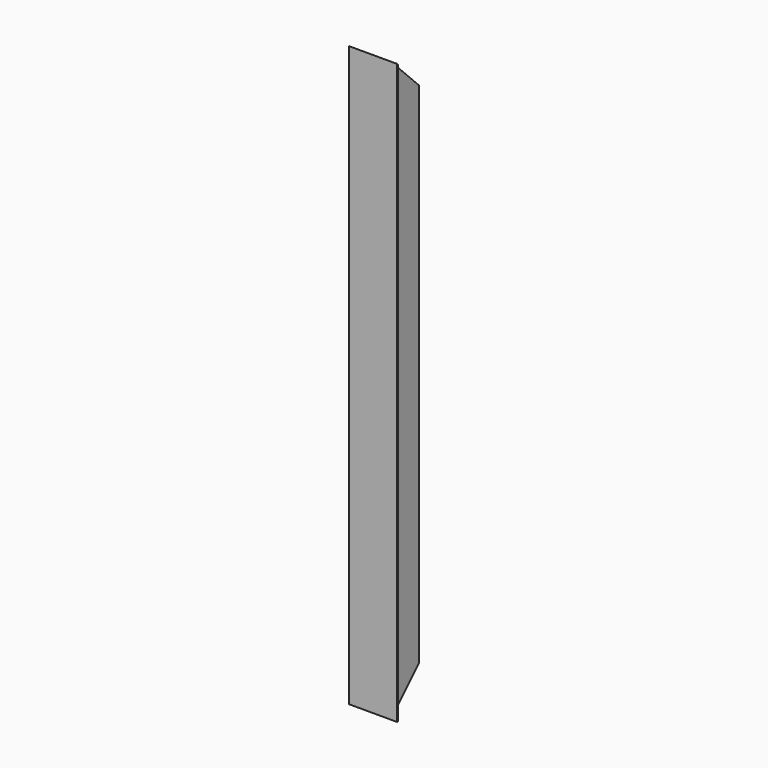
from build123d import *

# Parameters (mm, degrees)
F1_DEPTH = 228
F3_DEPTH = 30
F4_R     = 1
F6_R     = 0.5
F7_R     = 0.5


# Not quite as in the source:
# - two fillets or chamfers of one size are made in one step
# - a pattern or mirror of a feature is missing from the dataset's text; its kind, count and spacing are read off the source's solid


with BuildPart() as f1:
    # F0 (on Top) → F1 (new body, symmetric)
    with BuildSketch(Plane.XY):
        Polygon((-14, 0.5), (-17, 0.5), (-20, -2.5), (20, -2.5), (17, 0.5), (14, 0.5), (11, 0.5), (-11, 0.5), align=None)
        Polygon((-14, 25.5), (-14, 0.5), (-11, 0.5), (-11, 4), (-11, 7), (-11, 25.5), align=None)
        Polygon((11, 4), (11, 0.5), (14, 0.5), (14, 25.5), (11, 25.5), (11, 7), align=None)
        Polygon((-11, 7), (-11, 4), (-5, 4), (-5, 7), (-5, 15), (-8, 15), (-8, 7), align=None)
        Polygon((5, 4), (11, 4), (11, 7), (8, 7), (8, 15), (5, 15), (5, 7), align=None)
    extrude(amount=F1_DEPTH, both=True)

    # F2 (on Right) → F3 (cut, symmetric)
    with BuildSketch(Plane.YZ):
        Polygon((25.5, 228), (0.5, 228), (-2.5, 228), (25.5, 200), align=None)
    f3 = extrude(amount=F3_DEPTH, both=True, mode=Mode.SUBTRACT)

    # F3_copies: F3 across plane
    add(f3.mirror(Plane(origin=(0, 0, 0), x_dir=(-1, 0, 0), z_dir=(0, 0, -1))), mode=Mode.SUBTRACT)

    # F4
    f4_edges = [f1.edges().sort_by_distance(p)[0] for p in [
        (17, 0.5, 0),
        (12.5, 25.5, 200),
        (-11, 0.5, 0),
        (-12.5, 25.5, 200),
        (-17, 0.5, 0),
        (11, 0.5, 0),
        (6.5, 15, 210.5),
        (-6.5, 15, 210.5),
        (12.5, 25.5, -200),
        (6.5, 15, -210.5),
        (-6.5, 15, -210.5),
        (-12.5, 25.5, -200),
        (5, 4, 0),
        (-5, 4, 0),
    ]]
    fillet(f4_edges, radius=F4_R)

    # F6
    f6_edges = [f1.edges().sort_by_distance(p)[0] for p in [
        (8, 7, 0),
        (-11, 7, 0),
        (-11, 4, 0),
        (11, 4, 0),
        (11, 7, 0),
        (-8, 7, 0),
    ]]
    fillet(f6_edges, radius=F6_R)

    # F7
    f7_edges = [f1.edges().sort_by_distance(p)[0] for p in [
        (-20, -2.5, 0),
        (20, -2.5, 0),
        (14, 0.5, 0),
        (-14, 0.5, 0),
    ]]
    fillet(f7_edges, radius=F7_R)


solid = f1.part
